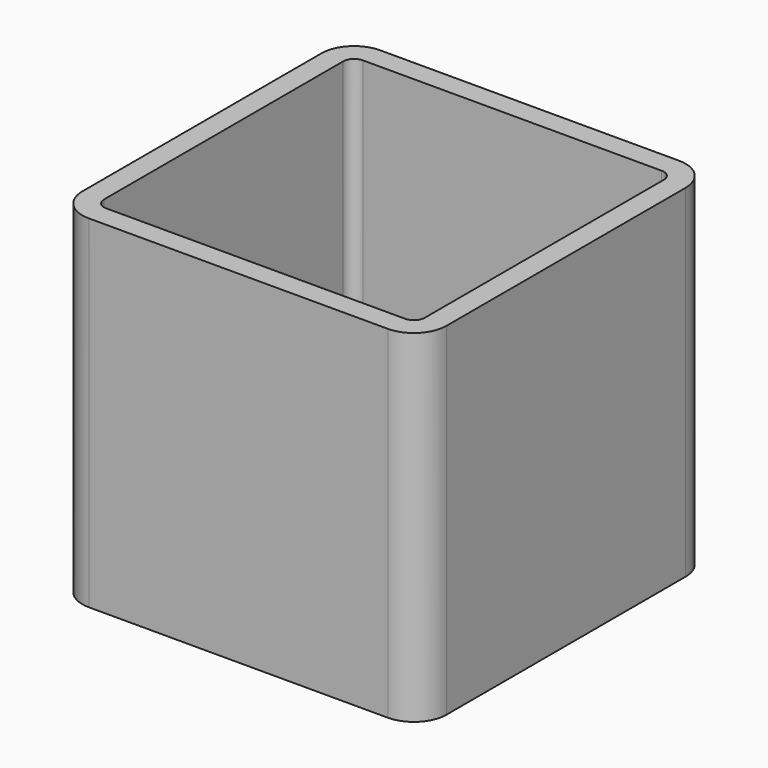
from build123d import *

# Parameters (mm, degrees)
F0_W     = 67
F0_H     = 67
F0_W_2   = 59
F0_H_2   = 59
F1_DEPTH = 4
F2_DEPTH = 63
F3_R     = 2
F4_R     = 6


with BuildPart() as f1:
    # F0 (on Top) → F1 (new body)
    with BuildSketch(Plane.XY):
        Rectangle(F0_W, F0_H)
        Rectangle(F0_W_2, F0_H_2, mode=Mode.SUBTRACT)
        Rectangle(F0_W_2, F0_H_2)
    extrude(amount=F1_DEPTH)

    # F0 (on Top) → F2 (join)
    with BuildSketch(Plane.XY):
        Rectangle(F0_W, F0_H)
        Rectangle(F0_W_2, F0_H_2, mode=Mode.SUBTRACT)
    extrude(amount=F2_DEPTH)

    # F3
    f3_edges = [f1.edges().sort_by_distance(p)[0] for p in [
        (29.5, -29.5, 33.5),
        (-29.5, -29.5, 33.5),
        (-29.5, 29.5, 33.5),
        (29.5, 29.5, 33.5),
        (-29.5, 0, 4),
        (0, 29.5, 4),
        (29.5, 0, 4),
        (0, -29.5, 4),
    ]]
    fillet(f3_edges, radius=F3_R)

    # F4
    f4_edges = [f1.edges().sort_by_distance(p)[0] for p in [
        (-33.5, 33.5, 31.5),
        (-33.5, -33.5, 31.5),
        (33.5, -33.5, 31.5),
        (33.5, 33.5, 31.5),
    ]]
    fillet(f4_edges, radius=F4_R)


solid = f1.part
